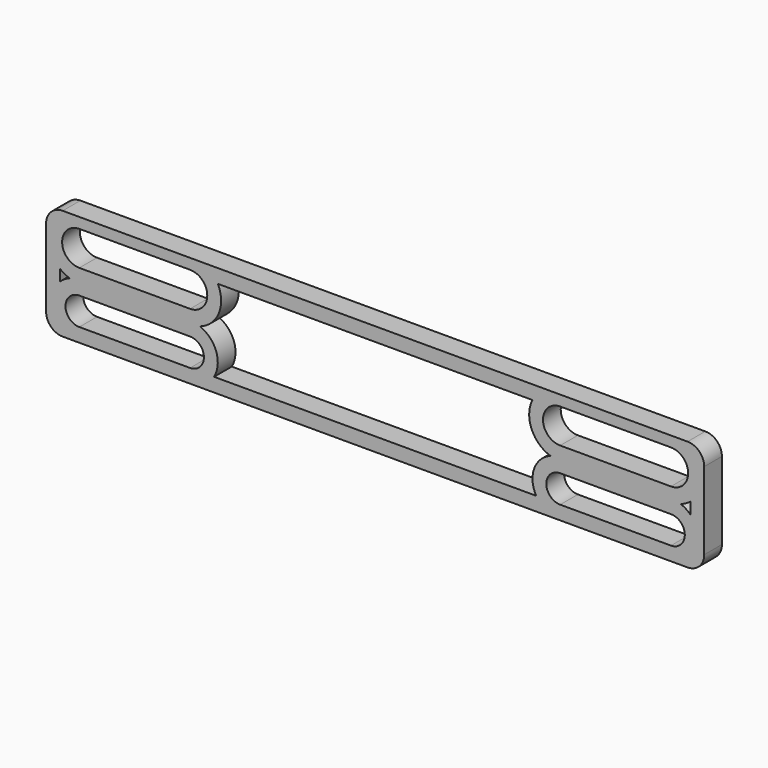
from build123d import *

# Parameters (mm, degrees)
F0_W     = 118.813
F0_H     = 20
F1_DEPTH = 4
F2_T     = 2.5
F3_R     = 3


# Not quite as in the source:
# - a shell that OpenCascade refuses in one call is made with other operations: the cavity is built on its own and cut out


with BuildPart() as f1:
    # F0 (on Front) → F1 (new body)
    with BuildSketch(Plane.XZ):
        Rectangle(F0_W, F0_H)
        with BuildLine():
            Line((-33.4065, -7.5), (-53.4065, -7.5))
            ThreePointArc((-53.4065, -7.5), (-55.9065, -5), (-53.4065, -2.5))
            Line((-53.4065, -2.5), (-33.4065, -2.5))
            ThreePointArc((-33.4065, -2.5), (-30.9065, -5), (-33.4065, -7.5))
        make_face(mode=Mode.SUBTRACT)
        with BuildLine():
            Line((53.4065, -7.5), (33.4065, -7.5))
            ThreePointArc((33.4065, -7.5), (30.9065, -5), (33.4065, -2.5))
            Line((33.4065, -2.5), (53.4065, -2.5))
            ThreePointArc((53.4065, -2.5), (55.9065, -5), (53.4065, -7.5))
        make_face(mode=Mode.SUBTRACT)
        with BuildLine():
            Line((-33.4065, 1.9), (-53.4065, 1.9))
            ThreePointArc((-53.4065, 1.9), (-56.5065, 5), (-53.4065, 8.1))
            Line((-53.4065, 8.1), (-33.4065, 8.1))
            ThreePointArc((-33.4065, 8.1), (-30.3065, 5), (-33.4065, 1.9))
        make_face(mode=Mode.SUBTRACT)
        with BuildLine():
            Line((53.4065, 1.9), (33.4065, 1.9))
            ThreePointArc((33.4065, 1.9), (30.3065, 5), (33.4065, 8.1))
            Line((33.4065, 8.1), (53.4065, 8.1))
            ThreePointArc((53.4065, 8.1), (56.5065, 5), (53.4065, 1.9))
        make_face(mode=Mode.SUBTRACT)
    extrude(amount=F1_DEPTH)

    # F2: shell of thickness 2.5, made by hand


with BuildPart() as f2_core1:
    # F2_t2: copy of F1
    add(f1.part)

    # the walls: a layer under each face that stays
    f2_faces = [f2_core1.faces().sort_by_distance(p)[0] for p in [
        (59.4065, -2, 0),
        (0, -2, 10),
        (-59.4065, -2, 0),
        (0, -2, -10),
        (-43.4065, -2, -7.5),
        (-55.9065, -2, -5),
        (-43.4065, -2, -2.5),
        (-30.9065, -2, -5),
        (43.4065, -2, -7.5),
        (30.9065, -2, -5),
        (43.4065, -2, -2.5),
        (55.9065, -2, -5),
        (-43.4065, -2, 8.1),
        (-30.3065, -2, 5),
        (-43.4065, -2, 1.9),
        (-56.5065, -2, 5),
        (43.4065, -2, 1.9),
        (30.3065, -2, 5),
        (43.4065, -2, 8.1),
        (56.5065, -2, 5),
    ]]
    thicken(f2_faces, amount=-F2_T, mode=Mode.SUBTRACT)


with BuildPart() as f1_1:
    add(f1.part)

    # what is left inside the walls is the cavity
    f2_cavity = [f2_core1.part.solids().sort_by_distance(p)[0] for p in [
        (56.105376, -2.666667, -0.761286),
        (0, -0.025, -2.5),
        (-56.105376, -2.666667, -0.761286),
    ]]
    add(f2_cavity, mode=Mode.SUBTRACT)

    # F3
    f3_edges = [f1_1.edges().sort_by_distance(p)[0] for p in [
        (59.4065, -2, -10),
        (59.4065, -2, 10),
        (-59.4065, -2, -10),
        (-59.4065, -2, 10),
    ]]
    fillet(f3_edges, radius=F3_R)


solid = f1_1.part
